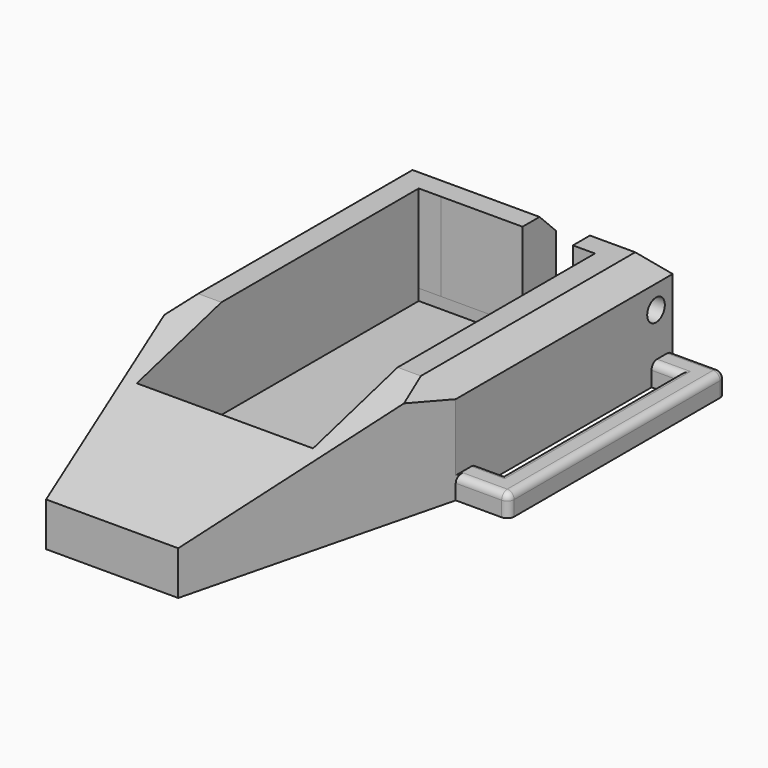
from build123d import *

# Parameters (mm, degrees)
F0_W        = 9.525
F0_H        = 13.4751944874
F0_W_2      = 3.175
F0_H_2      = 15.7348055126
F0_H_3      = 17.78
F0_H_4      = 3.81
F1_DEPTH    = 1.55575
F0_W_3      = 3.81
F0_H_5      = 31.4696110251
F0_W_4      = 6.35
F0_H_6      = 1.27
F0_H_7      = 19.05
F0_H_8      = 2.2596110251
F0_W_5      = 2.2601685487
F2_DEPTH    = 3.175
F3_R        = 1
F4_DEPTH    = 15.84325
F5_SIZE     = 3
F6_T1_DEPTH = 203.7288380727
F8_DEPTH    = 25.4


# Not quite as in the source:
# - a fillet or chamfer that OpenCascade refuses, or shapes differently, is made with other operations: its cross-section is extruded or revolved along the edge and cut away or added


with BuildPart() as f1:
    # F0 (on Top) → F1 (new body)
    with BuildSketch(Plane.XY):
        with Locations((-4.7625, 26.2824027563)):
            Rectangle(F0_W, F0_H)
        with Locations((-11.1125, 26.2824027563)):
            Rectangle(F0_W_2, F0_H)
        with Locations((-11.1125, 11.6774027563)):
            Rectangle(F0_W_2, F0_H_2)
        with Locations((-4.7625, 11.6774027563)):
            Rectangle(F0_W, F0_H_2)
        with Locations((4.7625, 11.6774027563)):
            Rectangle(F0_W, F0_H_2)
        with Locations((11.1125, 11.6774027563)):
            Rectangle(F0_W_2, F0_H_2)
        with Locations((11.1125, 26.2824027563)):
            Rectangle(F0_W_2, F0_H)
        Polygon((0, 33.02), (0, 19.5448055126), (9.525, 19.5448055126), (9.525, 33.02), (2.2601685487, 33.02), align=None)
        with Locations((-4.7625, -8.89)):
            Rectangle(F0_W, F0_H_3)
        with Locations((4.7625, -8.89)):
            Rectangle(F0_W, F0_H_3)
        with Locations((11.1125, -8.89)):
            Rectangle(F0_W_2, F0_H_3)
        with Locations((-11.1125, -8.89)):
            Rectangle(F0_W_2, F0_H_3)
        with Locations((-11.1125, 1.905)):
            Rectangle(F0_W_2, F0_H_4)
        with Locations((-4.7625, 1.905)):
            Rectangle(F0_W, F0_H_4)
        with Locations((4.7625, 1.905)):
            Rectangle(F0_W, F0_H_4)
        with Locations((11.1125, 1.905)):
            Rectangle(F0_W_2, F0_H_4)
    extrude(amount=F1_DEPTH)

    # F0 (on Top) → F2 (join)
    with BuildSketch(Plane.XY):
        Polygon((-12.7, 33.02), (-9.525, 33.02), (-9.525, 35.2796110251), (-19.05, 35.2796110251), (-19.05, 19.5448055126), (-12.7, 19.5448055126), align=None)
        with Locations((-14.2875, 37.1846110251)):
            Rectangle(F0_W, F0_H_4)
        with Locations((-20.955, 37.1846110251)):
            Rectangle(F0_W_3, F0_H_4)
        with Locations((-24.765, 37.1846110251)):
            Rectangle(F0_W_3, F0_H_4)
        with Locations((-24.765, 19.5448055126)):
            Rectangle(F0_W_3, F0_H_5)
        with Locations((-24.765, 1.905)):
            Rectangle(F0_W_3, F0_H_4)
        with Locations((-20.955, 1.905)):
            Rectangle(F0_W_3, F0_H_4)
        with Locations((-15.875, 1.905)):
            Rectangle(F0_W_4, F0_H_4)
        with Locations((-15.875, 11.6774027563)):
            Rectangle(F0_W_4, F0_H_2)
        Polygon((-9.525, -19.05), (-9.525, -17.78), (-12.7, -17.78), (-12.7, 0), (-19.05, 0), (-14.2875, -19.05), align=None)
        with Locations((-4.7625, -18.415)):
            Rectangle(F0_W, F0_H_6)
        with Locations((4.7625, -18.415)):
            Rectangle(F0_W, F0_H_6)
        Polygon((12.7, -17.78), (9.525, -17.78), (9.525, -19.05), (14.2875, -19.05), (19.05, 0), (12.7, 0), align=None)
        Polygon((14.2875, -19.05), (9.525, -19.05), (9.525, -38.1), align=None)
        Polygon((-9.525, -38.1), (-9.525, -19.05), (-14.2875, -19.05), align=None)
        with Locations((-4.7625, -28.575)):
            Rectangle(F0_W, F0_H_7)
        with Locations((4.7625, -28.575)):
            Rectangle(F0_W, F0_H_7)
        with Locations((15.875, 1.905)):
            Rectangle(F0_W_4, F0_H_4)
        with Locations((15.875, 11.6774027563)):
            Rectangle(F0_W_4, F0_H_2)
        Polygon((9.525, 35.2796110251), (9.525, 33.02), (12.7, 33.02), (12.7, 19.5448055126), (19.05, 19.5448055126), (19.05, 35.2796110251), align=None)
        with Locations((-4.7625, 34.1498055126)):
            Rectangle(F0_W, F0_H_8)
        with Locations((-4.7625, 37.1846110251)):
            Rectangle(F0_W, F0_H_4)
        with Locations((1.1300842743, 37.1846110251)):
            Rectangle(F0_W_5, F0_H_4)
        with Locations((14.2875, 37.1846110251)):
            Rectangle(F0_W, F0_H_4)
        with Locations((20.955, 37.1846110251)):
            Rectangle(F0_W_3, F0_H_4)
        with Locations((24.765, 37.1846110251)):
            Rectangle(F0_W_3, F0_H_4)
        with Locations((24.765, 19.5448055126)):
            Rectangle(F0_W_3, F0_H_5)
        with Locations((24.765, 1.905)):
            Rectangle(F0_W_3, F0_H_4)
        with Locations((20.955, 1.905)):
            Rectangle(F0_W_3, F0_H_4)
        with Locations((1.1300842743, 34.1498055126)):
            Rectangle(F0_W_5, F0_H_8)
    extrude(amount=F2_DEPTH)

    # F3
    f3_edges = [f1.edges().sort_by_distance(p)[0] for p in [
        (26.67, 19.544806, 3.175),
        (22.86, 0, 3.175),
        (26.67, 0, 1.5875),
        (26.67, 39.089611, 1.5875),
        (-12.204916, 39.089611, 3.175),
        (18.0975, 39.089611, 3.175),
        (20.955, 35.279611, 3.175),
        (20.955, 3.81, 3.175),
        (22.86, 19.544806, 3.175),
        (-26.67, 19.544806, 3.175),
        (-22.86, 0, 3.175),
        (-26.67, 0, 1.5875),
        (-22.86, 19.544806, 3.175),
        (-20.955, 35.279611, 3.175),
        (-26.67, 39.089611, 1.5875),
        (-20.955, 3.81, 3.175),
    ]]
    fillet(f3_edges, radius=F3_R)

    # F0 (on Top) → F4 (join)
    with BuildSketch(Plane.XY):
        with Locations((-14.2875, 37.1846110251)):
            Rectangle(F0_W, F0_H_4)
        Polygon((-12.7, 33.02), (-9.525, 33.02), (-9.525, 35.2796110251), (-19.05, 35.2796110251), (-19.05, 19.5448055126), (-12.7, 19.5448055126), align=None)
        with Locations((-4.7625, 34.1498055126)):
            Rectangle(F0_W, F0_H_8)
        with Locations((-4.7625, 37.1846110251)):
            Rectangle(F0_W, F0_H_4)
        with Locations((1.1300842743, 37.1846110251)):
            Rectangle(F0_W_5, F0_H_4)
        with Locations((1.1300842743, 34.1498055126)):
            Rectangle(F0_W_5, F0_H_8)
        with Locations((14.2875, 37.1846110251)):
            Rectangle(F0_W, F0_H_4)
        Polygon((9.525, 35.2796110251), (9.525, 33.02), (12.7, 33.02), (12.7, 19.5448055126), (19.05, 19.5448055126), (19.05, 35.2796110251), align=None)
        with Locations((15.875, 11.6774027563)):
            Rectangle(F0_W_4, F0_H_2)
        with Locations((15.875, 1.905)):
            Rectangle(F0_W_4, F0_H_4)
        Polygon((12.7, -17.78), (9.525, -17.78), (9.525, -19.05), (14.2875, -19.05), (19.05, 0), (12.7, 0), align=None)
        with Locations((4.7625, -18.415)):
            Rectangle(F0_W, F0_H_6)
        with Locations((-4.7625, -18.415)):
            Rectangle(F0_W, F0_H_6)
        Polygon((-9.525, -19.05), (-9.525, -17.78), (-12.7, -17.78), (-12.7, 0), (-19.05, 0), (-14.2875, -19.05), align=None)
        with Locations((-15.875, 11.6774027563)):
            Rectangle(F0_W_4, F0_H_2)
        with Locations((-15.875, 1.905)):
            Rectangle(F0_W_4, F0_H_4)
        Polygon((-9.525, -38.1), (-9.525, -19.05), (-14.2875, -19.05), align=None)
        Polygon((14.2875, -19.05), (9.525, -19.05), (9.525, -38.1), align=None)
        with Locations((4.7625, -28.575)):
            Rectangle(F0_W, F0_H_7)
        with Locations((-4.7625, -28.575)):
            Rectangle(F0_W, F0_H_7)
    extrude(amount=F4_DEPTH)

    # F5
    f5_edges = [f1.edges().sort_by_distance(p)[0] for p in [
        (-19.05, 19.544806, 15.84325),
        (-8.394916, 39.089611, 15.84325),
        (14.2875, 39.089611, 15.84325),
        (19.05, 19.544806, 15.84325),
    ]]
    chamfer(f5_edges, length=F5_SIZE)

    # F6: chamfer of 35.56 x 9.5282732829 on 1 edges, made by hand

    # F6_s2 → F6_t1 (cut)
    with BuildSketch(Plane.YZ.offset(-101.8644190363)):
        Polygon((-2.54, 15.84325), (-38.1, 6.3149767171), (-38.1, 15.84325), align=None)
    extrude(amount=F6_T1_DEPTH, mode=Mode.SUBTRACT)

    # F7 (on face) → F8 (cut)
    with BuildSketch(Plane(origin=(9.525, 0, 0), x_dir=(0, -1, 0), z_dir=(-1, 0, 0))):
        with BuildLine():
            ThreePointArc((-34.5021110251, 9.49325), (-34.96707901, 10.6157820151), (-36.0896110251, 11.08075))
            ThreePointArc((-36.0896110251, 11.08075), (-37.2121430402, 8.3707179849), (-34.5021110251, 9.49325))
        make_face()
    extrude(amount=-F8_DEPTH, mode=Mode.SUBTRACT)


solid = f1.part
